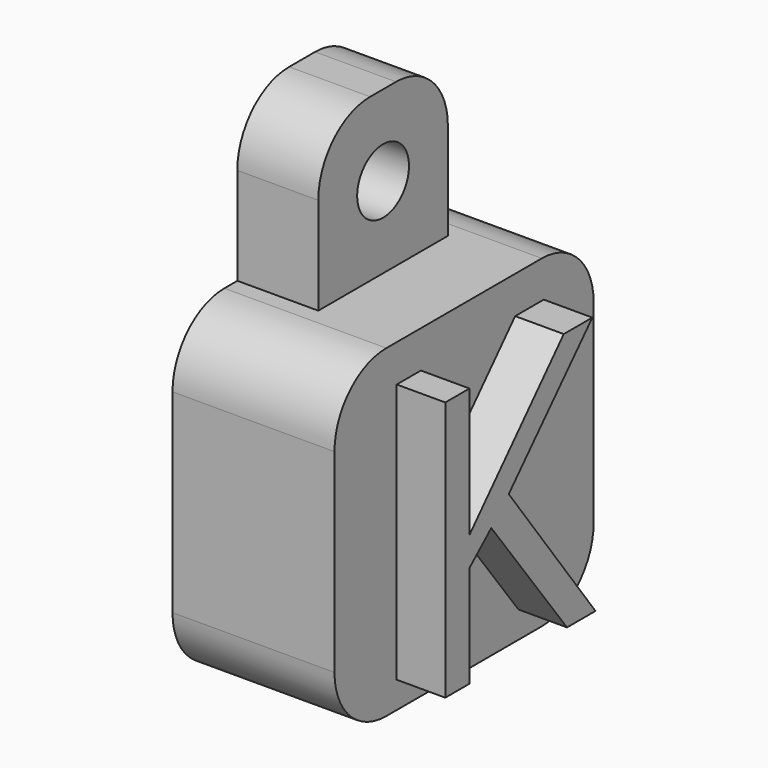
from build123d import *

# Parameters (mm, degrees)
F0_W          = 25.4
F0_H          = 25.4
F1_DEPTH      = 12.7
F2_W          = 12.7
F2_H          = 12.7
F3_DEPTH      = 6.35
F4_R          = 5.08
F5_R          = 5.08
F7_D          = 5.08
F8_R          = 5.08
F10_TEXT_SIZE = 28.5482823124
F11_DEPTH     = 3.81


# Not quite as in the source:
# - Text() gives the source's letters only with a copy of the font that has no kerning and outlines rounded to 1/6400 em; it was checked with that copy


with BuildPart() as f1:
    # F0 (on Right) → F1 (new body)
    with BuildSketch(Plane.YZ):
        Rectangle(F0_W, F0_H)
    extrude(amount=F1_DEPTH)

    # F8
    f8_edges = [f1.edges().sort_by_distance(p)[0] for p in [
        (6.35, -12.7, 12.7),
        (6.35, -12.7, -12.7),
        (6.35, 12.7, -12.7),
        (6.35, 12.7, 12.7),
    ]]
    fillet(f8_edges, radius=F8_R)

    # F10 (on face) → F11 (join)
    with BuildSketch(Plane.YZ.offset(12.7)):
        with Locations((-9.4022890553, -10.6053026393)):
            Text('K', F10_TEXT_SIZE, font='Open Sans', text_align=(TextAlign.LEFT, TextAlign.BOTTOM))
    extrude(amount=F11_DEPTH)


with BuildPart() as f3:
    # F2 (on Right) → F3 (new body)
    with BuildSketch(Plane.YZ):
        with Locations((0, 19.0536566079)):
            Rectangle(F2_W, F2_H)
    extrude(amount=F3_DEPTH)

    # F4
    f4_edges = [f3.edges().sort_by_distance(p)[0] for p in [
        (3.175, 6.35, 25.403657),
    ]]
    fillet(f4_edges, radius=F4_R)

    # F5
    f5_edges = [f3.edges().sort_by_distance(p)[0] for p in [
        (3.175, -6.35, 25.403657),
    ]]
    fillet(f5_edges, radius=F5_R)

    # F7 (through all)
    with Locations(Plane.YZ.offset(6.35)):
        with Locations((0, 19.0772153437)):
            Hole(F7_D / 2)


solid = Compound([f1.part, f3.part])
